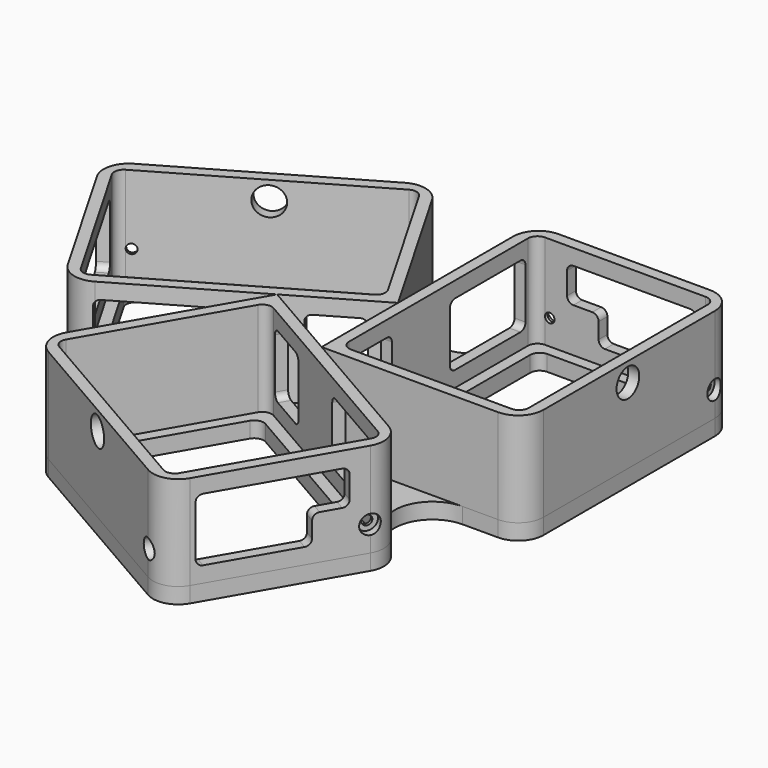
from build123d import *

# Parameters (mm, degrees)
F0_W                   = 57
F0_H                   = 77
F0_W_2                 = 50
F0_H_2                 = 70
F0_R                   = 6.25
F0_R_2                 = 3.25
F1_DEPTH               = 5
F2_DEPTH               = 2
F3_DEPTH               = 3
F4_DEPTH               = 30
F8_START               = -5
F7_W                   = 31
F7_H                   = 3.5
F7_W_2                 = 3.5
F7_H_2                 = 30
F7_H_3                 = 16
F8_DEPTH               = 20
F9_START               = -5
F7_W_3                 = 10
F9_DEPTH               = 11
F10_R                  = 4.5
F13_DEPTH              = 25
F12_R                  = 4.5
F14_DEPTH              = 25
F11_R                  = 4.5
F15_DEPTH              = 25
F23_D                  = 3
F23_DEPTH              = 12
F23_CBORE_D            = 6
F23_CBORE_DEPTH        = 2.5
F23_TIP                = 0.9012909285
F23_ON_F21_D           = 3
F23_ON_F21_DEPTH       = 12
F23_ON_F21_CBORE_D     = 6
F23_ON_F21_CBORE_DEPTH = 2.5
F23_ON_F21_TIP         = 0.9012909285
F23_ON_F20_D           = 3
F23_ON_F20_DEPTH       = 12
F23_ON_F20_CBORE_D     = 6
F23_ON_F20_CBORE_DEPTH = 2.5
F23_ON_F20_TIP         = 0.9012909285
F23_ON_F19_D           = 3
F23_ON_F19_DEPTH       = 12
F23_ON_F19_CBORE_D     = 6
F23_ON_F19_CBORE_DEPTH = 2.5
F23_ON_F19_TIP         = 0.9012909285
F23_ON_F18_D           = 3
F23_ON_F18_DEPTH       = 12
F23_ON_F18_CBORE_D     = 6
F23_ON_F18_CBORE_DEPTH = 2.5
F23_ON_F18_TIP         = 0.9012909285
F23_ON_F17_D           = 3
F23_ON_F17_DEPTH       = 12
F23_ON_F17_CBORE_D     = 6
F23_ON_F17_CBORE_DEPTH = 2.5
F23_ON_F17_TIP         = 0.9012909285
F24_F1_R               = 8
F24_F2_R               = 8
F24_F3_R               = 8
F24_F4_R               = 8
F24_F5_R               = 8
F24_F6_R               = 8
F24_F7_R               = 8
F24_F8_R               = 8
F24_F9_R               = 8
F24_2_T1_DEPTH         = 70
F24_3_T1_DEPTH         = 70
F24_4_T1_DEPTH         = 70
F25_R                  = 2.99999
F25_2_R                = 2.99999
F25_3_R                = 2.99999
F25_4_R                = 2.99999
F26_R                  = 2
F27_R                  = 2
F28_R                  = 2
F29_R                  = 12


# Not quite as in the source:
# - a fillet or chamfer that OpenCascade refuses, or shapes differently, is made with other operations: its cross-section is extruded or revolved along the edge and cut away or added
# - a fillet or chamfer is up to 0.001 mm smaller than in the source, because OpenCascade refuses the exact size
# - a feature names something its author has since deleted; it is built from what else it names


with BuildPart() as f1:
    # F0 (on Top) → F1 (new body)
    with BuildSketch(Plane.XY):
        Polygon((72.75, 68.8445554338), (8.75, 68.8445554338), (8.75, 15.1554445662), (8.75, -15.1554445662), (72.75, -15.1554445662), align=None)
        with Locations((40.75, 26.8445554338)):
            Rectangle(F0_W, F0_H, mode=Mode.SUBTRACT)
        Polygon((-17.5, 0), (8.75, 15.1554445662), (-23.25, 70.5810704084), (-95.9961339179, 28.5810704084), (-63.9961339179, -26.8445554338), align=None)
        Polygon((-62.7150450046, -22.0634665205), (-91.2150450046, 27.2999814952), (-24.5310889132, 65.7999814952), (3.9689110868, 16.4365334795), align=None, mode=Mode.SUBTRACT)
        Polygon((55.2461339179, -42), (8.75, -15.1554445662), (-17.5, 0), (-49.5, -55.4256258422), (23.2461339179, -97.4256258422), align=None)
        Polygon((21.9650450046, -92.644536929), (-44.7189110868, -54.144536929), (-16.2189110868, -4.7810889132), (50.4650450046, -43.2810889132), align=None, mode=Mode.SUBTRACT)
        with Locations((40.75, 26.8445554338)):
            Rectangle(F0_W, F0_H)
        with Locations((40.75, 26.8445554338)):
            Rectangle(F0_W_2, F0_H_2, mode=Mode.SUBTRACT)
        Polygon((-16.2189110868, -4.7810889132), (-44.7189110868, -54.144536929), (21.9650450046, -92.644536929), (50.4650450046, -43.2810889132), align=None)
        Polygon((20.6839560914, -87.8634480157), (-39.9378221735, -52.8634480157), (-14.9378221735, -9.5621778265), (45.6839560914, -44.5621778265), align=None, mode=Mode.SUBTRACT)
        Polygon((-24.5310889132, 65.7999814952), (-91.2150450046, 27.2999814952), (-62.7150450046, -22.0634665205), (3.9689110868, 16.4365334795), align=None)
        Polygon((-61.4339560914, -17.2823776073), (-86.4339560914, 26.0188925819), (-25.8121778265, 61.0188925819), (-0.8121778265, 17.7176223927), align=None, mode=Mode.SUBTRACT)
        Polygon((8.75, -15.1554445662), (8.75, 15.1554445662), (-17.5, 0), align=None)
        Circle(F0_R, mode=Mode.SUBTRACT)
        Circle(F0_R)
        Circle(F0_R_2, mode=Mode.SUBTRACT)
    extrude(amount=-F1_DEPTH)

    # F0 (on Top) → F2 (cut)
    with BuildSketch(Plane.XY):
        Circle(F0_R)
        Circle(F0_R_2, mode=Mode.SUBTRACT)
    extrude(amount=-F2_DEPTH, mode=Mode.SUBTRACT)

    # F0 (on Top) → F3 (cut)
    with BuildSketch(Plane.XY):
        with Locations((40.75, 26.8445554338)):
            Rectangle(F0_W, F0_H)
        with Locations((40.75, 26.8445554338)):
            Rectangle(F0_W_2, F0_H_2, mode=Mode.SUBTRACT)
        Polygon((-16.2189110868, -4.7810889132), (-44.7189110868, -54.144536929), (21.9650450046, -92.644536929), (50.4650450046, -43.2810889132), align=None)
        Polygon((20.6839560914, -87.8634480157), (-39.9378221735, -52.8634480157), (-14.9378221735, -9.5621778265), (45.6839560914, -44.5621778265), align=None, mode=Mode.SUBTRACT)
    extrude(amount=F3_DEPTH, mode=Mode.SUBTRACT)

    # F24: fillet of radius 8 on 9 edges, made by hand

    # F24_f1
    f24_f1_edges = [f1.edges().sort_by_distance(p)[0] for p in [
        (72.75, -15.1554445662, -2.5),
    ]]
    fillet(f24_f1_edges, radius=F24_F1_R)

    # F24_f2
    f24_f2_edges = [f1.edges().sort_by_distance(p)[0] for p in [
        (55.2461339179, -42, -2.5),
    ]]
    fillet(f24_f2_edges, radius=F24_F2_R)

    # F24_f3
    f24_f3_edges = [f1.edges().sort_by_distance(p)[0] for p in [
        (72.75, 68.8445554338, -2.5),
    ]]
    fillet(f24_f3_edges, radius=F24_F3_R)

    # F24_f4
    f24_f4_edges = [f1.edges().sort_by_distance(p)[0] for p in [
        (23.2461339179, -97.4256258422, -2.5),
    ]]
    fillet(f24_f4_edges, radius=F24_F4_R)

    # F24_f5
    f24_f5_edges = [f1.edges().sort_by_distance(p)[0] for p in [
        (8.75, 68.8445554338, -2.5),
    ]]
    fillet(f24_f5_edges, radius=F24_F5_R)

    # F24_f6
    f24_f6_edges = [f1.edges().sort_by_distance(p)[0] for p in [
        (-49.5, -55.4256258422, -2.5),
    ]]
    fillet(f24_f6_edges, radius=F24_F6_R)

    # F24_f7
    f24_f7_edges = [f1.edges().sort_by_distance(p)[0] for p in [
        (-23.25, 70.5810704084, -2.5),
    ]]
    fillet(f24_f7_edges, radius=F24_F7_R)

    # F24_f8
    f24_f8_edges = [f1.edges().sort_by_distance(p)[0] for p in [
        (-63.9961339179, -26.8445554338, -2.5),
    ]]
    fillet(f24_f8_edges, radius=F24_F8_R)

    # F24_f9
    f24_f9_edges = [f1.edges().sort_by_distance(p)[0] for p in [
        (-95.9961339179, 28.5810704084, -2.5),
    ]]
    fillet(f24_f9_edges, radius=F24_F9_R)

    # F25 (radius 3 in the source; OpenCascade refuses exactly that, so slightly less here)
    f25_edges = [f1.edges().sort_by_distance(p)[0] for p in [
        (-39.937822, -52.863448, -2.5),
        (15.75, 61.844555, -2.5),
        (15.75, -8.155445, -2.5),
        (20.683956, -87.863448, -2.5),
        (65.75, -8.155445, -2.5),
        (45.683956, -44.562178, -2.5),
        (65.75, 61.844555, -2.5),
        (-14.937822, -9.562178, -2.5),
        (-25.812178, 61.018893, -2.5),
        (-86.433956, 26.018893, -2.5),
        (-0.812178, 17.717622, -2.5),
        (-61.433956, -17.282378, -2.5),
    ]]
    fillet(f25_edges, radius=F25_R)

    # F29
    f29_edges = [f1.edges().sort_by_distance(p)[0] for p in [
        (8.75, -15.155445, -2.5),
        (8.75, 15.155445, -2.5),
        (-17.5, 0, -2.5),
    ]]
    fillet(f29_edges, radius=F29_R)


with BuildPart() as f4:
    # F0 (on Top) → F4 (new body)
    with BuildSketch(Plane.XY):
        Polygon((72.75, 68.8445554338), (8.75, 68.8445554338), (8.75, 15.1554445662), (8.75, -15.1554445662), (72.75, -15.1554445662), align=None)
        with Locations((40.75, 26.8445554338)):
            Rectangle(F0_W, F0_H, mode=Mode.SUBTRACT)
    extrude(amount=F4_DEPTH)


with BuildPart() as f4b:
    # F0 (on Top) → F4, piece 2 (new body)
    with BuildSketch(Plane.XY):
        Polygon((55.2461339179, -42), (8.75, -15.1554445662), (-17.5, 0), (-49.5, -55.4256258422), (23.2461339179, -97.4256258422), align=None)
        Polygon((21.9650450046, -92.644536929), (-44.7189110868, -54.144536929), (-16.2189110868, -4.7810889132), (50.4650450046, -43.2810889132), align=None, mode=Mode.SUBTRACT)
    extrude(amount=F4_DEPTH)


with BuildPart() as f4c:
    # F0 (on Top) → F4, piece 3 (new body)
    with BuildSketch(Plane.XY):
        Polygon((-17.5, 0), (8.75, 15.1554445662), (-23.25, 70.5810704084), (-95.9961339179, 28.5810704084), (-63.9961339179, -26.8445554338), align=None)
        Polygon((-62.7150450046, -22.0634665205), (-91.2150450046, 27.2999814952), (-24.5310889132, 65.7999814952), (3.9689110868, 16.4365334795), align=None, mode=Mode.SUBTRACT)
    extrude(amount=F4_DEPTH)


with BuildPart() as f8_tool:
    # F6 (on face) + F7 (on face) + F5 (on face) → F8 (new body)
    with BuildSketch(Plane.XY.offset(30).offset(F8_START)):
        Polygon((40.4650450046, -60.6015969889), (24.9650450046, -87.4483845063), (27.9961339179, -89.1983845063), (43.4961339179, -62.3515969889), align=None)
        Polygon((21.020181276, -26.2810889132), (47.0009433895, -41.2810889132), (48.7509433895, -38.25), (22.770181276, -23.25), align=None)
        Polygon((-11.0048094716, -3.75), (-12.7548094716, -6.7810889132), (1.1015969889, -14.7810889132), (2.8515969889, -11.75), align=None)
    with BuildSketch(Plane.XY.offset(30).offset(F8_START)):
        with Locations((47.75, 67.0945554338)):
            Rectangle(F7_W, F7_H)
        with Locations((10.5, 46.3445554338)):
            Rectangle(F7_W_2, F7_H_2)
        with Locations((10.5, 0.3445554338)):
            Rectangle(F7_W_2, F7_H_3)
    with BuildSketch(Plane.XY.offset(30).offset(F8_START)):
        Polygon((-88.2150450046, 22.1038290725), (-91.2461339179, 20.3538290725), (-75.7461339179, -6.4929584448), (-72.7150450046, -4.7429584448), align=None)
        Polygon((-59.2509433895, -20.0634665205), (-57.5009433895, -23.0945554338), (-31.520181276, -8.0945554338), (-33.270181276, -5.0634665205), align=None)
        Polygon((-11.6015969889, 3.4054445662), (2.2548094716, 11.4054445662), (0.5048094716, 14.4365334795), (-13.3515969889, 6.4365334795), align=None)
    extrude(amount=-F8_DEPTH)


with BuildPart() as f4_1:
    add(f4.part)

    # F8: cut by f8_tool
    add(f8_tool.part, mode=Mode.SUBTRACT)


with BuildPart() as f4b_1:
    add(f4b.part)

    # F8: cut by f8_tool
    add(f8_tool.part, mode=Mode.SUBTRACT)


with BuildPart() as f4c_1:
    add(f4c.part)

    # F8: cut by f8_tool
    add(f8_tool.part, mode=Mode.SUBTRACT)


with BuildPart() as f9_tool:
    # F5 (on face) + F6 (on face) + F7 (on face) → F9 (new body)
    with BuildSketch(Plane.XY.offset(30).offset(F9_START)):
        Polygon((-72.7150450046, -4.7429584448), (-75.7461339179, -6.4929584448), (-70.7461339179, -15.1532124827), (-67.7150450046, -13.4032124827), align=None)
    with BuildSketch(Plane.XY.offset(30).offset(F9_START)):
        Polygon((45.4650450046, -51.9413429511), (40.4650450046, -60.6015969889), (43.4961339179, -62.3515969889), (48.4961339179, -53.6913429511), align=None)
    with BuildSketch(Plane.XY.offset(30).offset(F9_START)):
        with Locations((27.25, 67.0945554338)):
            Rectangle(F7_W_3, F7_H)
    extrude(amount=-F9_DEPTH)


with BuildPart() as f4_2:
    add(f4_1.part)

    # F9: cut by f9_tool
    add(f9_tool.part, mode=Mode.SUBTRACT)

    # F11 (on face) → F15 (cut)
    with BuildSketch(Plane.YZ.offset(72.75)):
        with Locations((26.3445554338, 24)):
            Circle(F11_R)
    extrude(amount=-F15_DEPTH, mode=Mode.SUBTRACT)

    # F23 on F20
    with Locations(Plane(origin=(0, 68.8445554338, 0), x_dir=(-1, 0, 0), z_dir=(0, 1, 0))):
        with Locations((-16.75, 8)):
            CounterBoreHole(F23_ON_F20_D / 2, F23_ON_F20_CBORE_D / 2, F23_ON_F20_CBORE_DEPTH, depth=F23_ON_F20_DEPTH)
            with Locations((0, 0, -(F23_ON_F20_DEPTH + F23_ON_F20_TIP / 2))):  # 118° drill point
                Cone(0, F23_ON_F20_D / 2, F23_ON_F20_TIP, mode=Mode.SUBTRACT)

    # F23 on F19
    with Locations(Plane.YZ.offset(72.75)):
        with Locations((60.8445554338, 8)):
            CounterBoreHole(F23_ON_F19_D / 2, F23_ON_F19_CBORE_D / 2, F23_ON_F19_CBORE_DEPTH, depth=F23_ON_F19_DEPTH)
            with Locations((0, 0, -(F23_ON_F19_DEPTH + F23_ON_F19_TIP / 2))):  # 118° drill point
                Cone(0, F23_ON_F19_D / 2, F23_ON_F19_TIP, mode=Mode.SUBTRACT)

    # F24#2: fillet of radius 8 on 3 edges, made by hand

    # F24_2_s2 → F24_2_t1 (cut)
    with BuildSketch(Plane.XY.offset(-20)):
        with BuildLine():
            ThreePointArc((72.75, 60.8445554338), (70.4068542495, 66.5014096833), (64.75, 68.8445554338))
            Line((64.75, 68.8445554338), (72.75, 68.8445554338))
            Line((72.75, 68.8445554338), (72.75, 60.8445554338))
        make_face()
        with BuildLine():
            ThreePointArc((16.75, 68.8445554338), (11.0931457505, 66.5014096833), (8.75, 60.8445554338))
            Line((8.75, 60.8445554338), (8.75, 68.8445554338))
            Line((8.75, 68.8445554338), (16.75, 68.8445554338))
        make_face()
        with BuildLine():
            ThreePointArc((72.75, -7.1554445662), (70.4068542495, -12.8122988157), (64.75, -15.1554445662))
            Line((64.75, -15.1554445662), (72.75, -15.1554445662))
            Line((72.75, -15.1554445662), (72.75, -7.1554445662))
        make_face()
    extrude(amount=F24_2_T1_DEPTH, mode=Mode.SUBTRACT)

    # F25#2 (radius 3 in the source; OpenCascade refuses exactly that, so slightly less here)
    f25_2_edges = [f4_2.edges().sort_by_distance(p)[0] for p in [
        (69.25, -11.655445, 15),
        (69.25, 65.344555, 15),
        (12.25, 65.344555, 15),
        (12.25, -11.655445, 15),
    ]]
    fillet(f25_2_edges, radius=F25_2_R)

    # F26 (call 1 of 14: OpenCascade refuses the feature's edges together)
    f26_edges = [f4_2.edges().sort_by_distance(p)[0] for p in [
        (32.25, 67.094555, 5),
    ]]
    fillet(f26_edges, radius=F26_R)

    # F26#2 (call 2 of 14)
    f26_2_edges = [f4_2.edges().sort_by_distance(p)[0] for p in [
        (22.25, 67.094555, 14),
    ]]
    fillet(f26_2_edges, radius=F26_R)

    # F26#3 (call 3 of 14)
    f26_3_edges = [f4_2.edges().sort_by_distance(p)[0] for p in [
        (32.25, 67.094555, 14),
    ]]
    fillet(f26_3_edges, radius=F26_R)

    # F26#4 (call 4 of 14)
    f26_4_edges = [f4_2.edges().sort_by_distance(p)[0] for p in [
        (63.25, 67.094555, 5),
    ]]
    fillet(f26_4_edges, radius=F26_R)

    # F26#5 (call 5 of 14)
    f26_5_edges = [f4_2.edges().sort_by_distance(p)[0] for p in [
        (63.25, 67.094555, 25),
    ]]
    fillet(f26_5_edges, radius=F26_R)

    # F26#6 (call 6 of 14)
    f26_6_edges = [f4_2.edges().sort_by_distance(p)[0] for p in [
        (22.25, 67.094555, 25),
    ]]
    fillet(f26_6_edges, radius=F26_R)

    # F26#7 (call 7 of 14)
    f26_7_edges = [f4_2.edges().sort_by_distance(p)[0] for p in [
        (10.50782, 61.344555, 5),
    ]]
    fillet(f26_7_edges, radius=F26_R)

    # F26#8 (call 8 of 14)
    f26_8_edges = [f4_2.edges().sort_by_distance(p)[0] for p in [
        (10.5, 31.344555, 5),
    ]]
    fillet(f26_8_edges, radius=F26_R)

    # F26#9 (call 9 of 14)
    f26_9_edges = [f4_2.edges().sort_by_distance(p)[0] for p in [
        (10.5, 31.344555, 25),
    ]]
    fillet(f26_9_edges, radius=F26_R)

    # F26#10 (call 10 of 14)
    f26_10_edges = [f4_2.edges().sort_by_distance(p)[0] for p in [
        (10.50782, 61.344555, 25),
    ]]
    fillet(f26_10_edges, radius=F26_R)

    # F26#11 (call 11 of 14)
    f26_11_edges = [f4_2.edges().sort_by_distance(p)[0] for p in [
        (10.5, -7.655445, 5),
    ]]
    fillet(f26_11_edges, radius=F26_R)

    # F26#12 (call 12 of 14)
    f26_12_edges = [f4_2.edges().sort_by_distance(p)[0] for p in [
        (10.5, 8.344555, 5),
    ]]
    fillet(f26_12_edges, radius=F26_R)

    # F26#13 (call 13 of 14)
    f26_13_edges = [f4_2.edges().sort_by_distance(p)[0] for p in [
        (10.5, 8.344555, 25),
    ]]
    fillet(f26_13_edges, radius=F26_R)

    # F26#14 (call 14 of 14)
    f26_14_edges = [f4_2.edges().sort_by_distance(p)[0] for p in [
        (10.5, -7.655445, 25),
    ]]
    fillet(f26_14_edges, radius=F26_R)


with BuildPart() as f4b_2:
    add(f4b_1.part)

    # F9: cut by f9_tool
    add(f9_tool.part, mode=Mode.SUBTRACT)

    # F10 (on face) → F13 (cut)
    with BuildSketch(Plane(origin=(-36.375, -63.0033481253, 0), x_dir=(0.8660254038, -0.5, 0), z_dir=(-0.5, -0.8660254038, 0))):
        with Locations((26.3445554338, 24)):
            Circle(F10_R)
    extrude(amount=-F13_DEPTH, mode=Mode.SUBTRACT)

    # F23 on F18
    with Locations(Plane(origin=(59.6211339179, -34.4222777169, 0), x_dir=(0.5, 0.8660254038, 0), z_dir=(0.8660254038, -0.5, 0))):
        with Locations((-16.75, 8)):
            CounterBoreHole(F23_ON_F18_D / 2, F23_ON_F18_CBORE_D / 2, F23_ON_F18_CBORE_DEPTH, depth=F23_ON_F18_DEPTH)
            with Locations((0, 0, -(F23_ON_F18_DEPTH + F23_ON_F18_TIP / 2))):  # 118° drill point
                Cone(0, F23_ON_F18_D / 2, F23_ON_F18_TIP, mode=Mode.SUBTRACT)

    # F23 on F17
    with Locations(Plane(origin=(-36.375, -63.0033481253, 0), x_dir=(0.8660254038, -0.5, 0), z_dir=(-0.5, -0.8660254038, 0))):
        with Locations((60.8445554338, 8)):
            CounterBoreHole(F23_ON_F17_D / 2, F23_ON_F17_CBORE_D / 2, F23_ON_F17_CBORE_DEPTH, depth=F23_ON_F17_DEPTH)
            with Locations((0, 0, -(F23_ON_F17_DEPTH + F23_ON_F17_TIP / 2))):  # 118° drill point
                Cone(0, F23_ON_F17_D / 2, F23_ON_F17_TIP, mode=Mode.SUBTRACT)

    # F24#3: fillet of radius 8 on 3 edges, made by hand

    # F24_3_s2 → F24_3_t1 (cut)
    with BuildSketch(Plane.XY.offset(-20)):
        with BuildLine():
            ThreePointArc((-42.5717967697, -59.4256258422), (-46.29920338, -54.5679749727), (-45.5, -48.4974226119))
            Line((-45.5, -48.4974226119), (-49.5, -55.4256258422))
            Line((-49.5, -55.4256258422), (-42.5717967697, -59.4256258422))
        make_face()
        with BuildLine():
            ThreePointArc((27.2461339179, -90.4974226119), (22.3884830484, -94.2248292222), (16.3179306876, -93.4256258422))
            Line((16.3179306876, -93.4256258422), (23.2461339179, -97.4256258422))
            Line((23.2461339179, -97.4256258422), (27.2461339179, -90.4974226119))
        make_face()
        with BuildLine():
            ThreePointArc((51.2461339179, -48.9282032303), (52.0453372979, -42.8576508695), (48.3179306876, -38))
            Line((48.3179306876, -38), (55.2461339179, -42))
            Line((55.2461339179, -42), (51.2461339179, -48.9282032303))
        make_face()
    extrude(amount=F24_3_T1_DEPTH, mode=Mode.SUBTRACT)

    # F25#3 (radius 3 in the source; OpenCascade refuses exactly that, so slightly less here)
    f25_3_edges = [f4b_2.edges().sort_by_distance(p)[0] for p in [
        (50.465045, -43.281089, 15),
        (21.965045, -92.644537, 15),
        (-16.218911, -4.781089, 15),
        (-44.718911, -54.144537, 15),
    ]]
    fillet(f25_3_edges, radius=F25_3_R)

    # F28
    f28_edges = [f4b_2.edges().sort_by_distance(p)[0] for p in [
        (26.480589, -88.323385, 5),
        (21.895181, -24.765544, 5),
        (-11.879809, -5.265544, 5),
        (41.980589, -61.476597, 14),
        (46.980589, -52.816343, 14),
        (46.980589, -52.816343, 25),
        (21.895181, -24.765544, 25),
        (-11.879809, -5.265544, 25),
        (47.872033, -39.772317, 25),
        (1.976597, -13.265544, 25),
        (47.872033, -39.772317, 5),
        (1.976597, -13.265544, 5),
        (26.480589, -88.323385, 25),
        (41.980589, -61.476597, 5),
    ]]
    fillet(f28_edges, radius=F28_R)


with BuildPart() as f4c_2:
    add(f4c_1.part)

    # F9: cut by f9_tool
    add(f9_tool.part, mode=Mode.SUBTRACT)

    # F12 (on face) → F14 (cut)
    with BuildSketch(Plane(origin=(-36.375, 63.0033481253, 0), x_dir=(-0.8660254038, -0.5, 0), z_dir=(-0.5, 0.8660254038, 0))):
        with Locations((26.3445554338, 24)):
            Circle(F12_R)
    extrude(amount=-F14_DEPTH, mode=Mode.SUBTRACT)

    # F23
    with Locations(Plane(origin=(-59.6211339179, -34.4222777169, 0), x_dir=(0.5, -0.8660254038, 0), z_dir=(-0.8660254038, -0.5, 0))):
        with Locations((-16.75, 8)):
            CounterBoreHole(F23_D / 2, F23_CBORE_D / 2, F23_CBORE_DEPTH, depth=F23_DEPTH)
            with Locations((0, 0, -(F23_DEPTH + F23_TIP / 2))):  # 118° drill point
                Cone(0, F23_D / 2, F23_TIP, mode=Mode.SUBTRACT)

    # F23 on F21
    with Locations(Plane(origin=(-36.375, 63.0033481253, 0), x_dir=(-0.8660254038, -0.5, 0), z_dir=(-0.5, 0.8660254038, 0))):
        with Locations((60.8445554338, 8)):
            CounterBoreHole(F23_ON_F21_D / 2, F23_ON_F21_CBORE_D / 2, F23_ON_F21_CBORE_DEPTH, depth=F23_ON_F21_DEPTH)
            with Locations((0, 0, -(F23_ON_F21_DEPTH + F23_ON_F21_TIP / 2))):  # 118° drill point
                Cone(0, F23_ON_F21_D / 2, F23_ON_F21_TIP, mode=Mode.SUBTRACT)

    # F24#4: fillet of radius 8 on 3 edges, made by hand

    # F24_4_s2 → F24_4_t1 (cut)
    with BuildSketch(Plane.XY.offset(-20)):
        with BuildLine():
            ThreePointArc((-19.25, 63.6528671782), (-24.1076508695, 67.3802737885), (-30.1782032303, 66.5810704084))
            Line((-30.1782032303, 66.5810704084), (-23.25, 70.5810704084))
            Line((-23.25, 70.5810704084), (-19.25, 63.6528671782))
        make_face()
        with BuildLine():
            ThreePointArc((-91.9961339179, 21.6528671782), (-92.7953372979, 27.723419539), (-89.0679306876, 32.5810704084))
            Line((-89.0679306876, 32.5810704084), (-95.9961339179, 28.5810704084))
            Line((-95.9961339179, 28.5810704084), (-91.9961339179, 21.6528671782))
        make_face()
        with BuildLine():
            ThreePointArc((-57.0679306876, -22.8445554338), (-63.1384830484, -23.6437588138), (-67.9961339179, -19.9163522035))
            Line((-67.9961339179, -19.9163522035), (-63.9961339179, -26.8445554338))
            Line((-63.9961339179, -26.8445554338), (-57.0679306876, -22.8445554338))
        make_face()
    extrude(amount=F24_4_T1_DEPTH, mode=Mode.SUBTRACT)

    # F25#4 (radius 3 in the source; OpenCascade refuses exactly that, so slightly less here)
    f25_4_edges = [f4c_2.edges().sort_by_distance(p)[0] for p in [
        (-91.215045, 27.299981, 15),
        (-24.531089, 65.799981, 15),
        (-62.715045, -22.063467, 15),
        (3.968911, 16.436533, 15),
    ]]
    fillet(f25_4_edges, radius=F25_4_R)

    # F27 (call 1 of 14: OpenCascade refuses the feature's edges together)
    f27_edges = [f4c_2.edges().sort_by_distance(p)[0] for p in [
        (1.379809, 12.920989, 5),
    ]]
    fillet(f27_edges, radius=F27_R)

    # F27#2 (call 2 of 14)
    f27_2_edges = [f4c_2.edges().sort_by_distance(p)[0] for p in [
        (-12.476597, 4.920989, 5),
    ]]
    fillet(f27_2_edges, radius=F27_R)

    # F27#3 (call 3 of 14)
    f27_3_edges = [f4c_2.edges().sort_by_distance(p)[0] for p in [
        (1.379809, 12.920989, 25),
    ]]
    fillet(f27_3_edges, radius=F27_R)

    # F27#4 (call 4 of 14)
    f27_4_edges = [f4c_2.edges().sort_by_distance(p)[0] for p in [
        (-12.476597, 4.920989, 25),
    ]]
    fillet(f27_4_edges, radius=F27_R)

    # F27#5 (call 5 of 14)
    f27_5_edges = [f4c_2.edges().sort_by_distance(p)[0] for p in [
        (-58.379853, -21.572239, 25),
    ]]
    fillet(f27_5_edges, radius=F27_R)

    # F27#6 (call 6 of 14)
    f27_6_edges = [f4c_2.edges().sort_by_distance(p)[0] for p in [
        (-32.395181, -6.579011, 25),
    ]]
    fillet(f27_6_edges, radius=F27_R)

    # F27#7 (call 7 of 14)
    f27_7_edges = [f4c_2.edges().sort_by_distance(p)[0] for p in [
        (-32.395181, -6.579011, 5),
    ]]
    fillet(f27_7_edges, radius=F27_R)

    # F27#8 (call 8 of 14)
    f27_8_edges = [f4c_2.edges().sort_by_distance(p)[0] for p in [
        (-58.379853, -21.572239, 5),
    ]]
    fillet(f27_8_edges, radius=F27_R)

    # F27#9 (call 9 of 14)
    f27_9_edges = [f4c_2.edges().sort_by_distance(p)[0] for p in [
        (-74.230589, -5.617958, 5),
    ]]
    fillet(f27_9_edges, radius=F27_R)

    # F27#10 (call 10 of 14)
    f27_10_edges = [f4c_2.edges().sort_by_distance(p)[0] for p in [
        (-69.230589, -14.278212, 14),
    ]]
    fillet(f27_10_edges, radius=F27_R)

    # F27#11 (call 11 of 14)
    f27_11_edges = [f4c_2.edges().sort_by_distance(p)[0] for p in [
        (-74.230589, -5.617958, 14),
    ]]
    fillet(f27_11_edges, radius=F27_R)

    # F27#12 (call 12 of 14)
    f27_12_edges = [f4c_2.edges().sort_by_distance(p)[0] for p in [
        (-69.230589, -14.278212, 25),
    ]]
    fillet(f27_12_edges, radius=F27_R)

    # F27#13 (call 13 of 14)
    f27_13_edges = [f4c_2.edges().sort_by_distance(p)[0] for p in [
        (-89.730589, 21.228829, 25),
    ]]
    fillet(f27_13_edges, radius=F27_R)

    # F27#14 (call 14 of 14)
    f27_14_edges = [f4c_2.edges().sort_by_distance(p)[0] for p in [
        (-89.730589, 21.228829, 5),
    ]]
    fillet(f27_14_edges, radius=F27_R)


solid = Compound([f1.part, f4_2.part, f4b_2.part, f4c_2.part])
